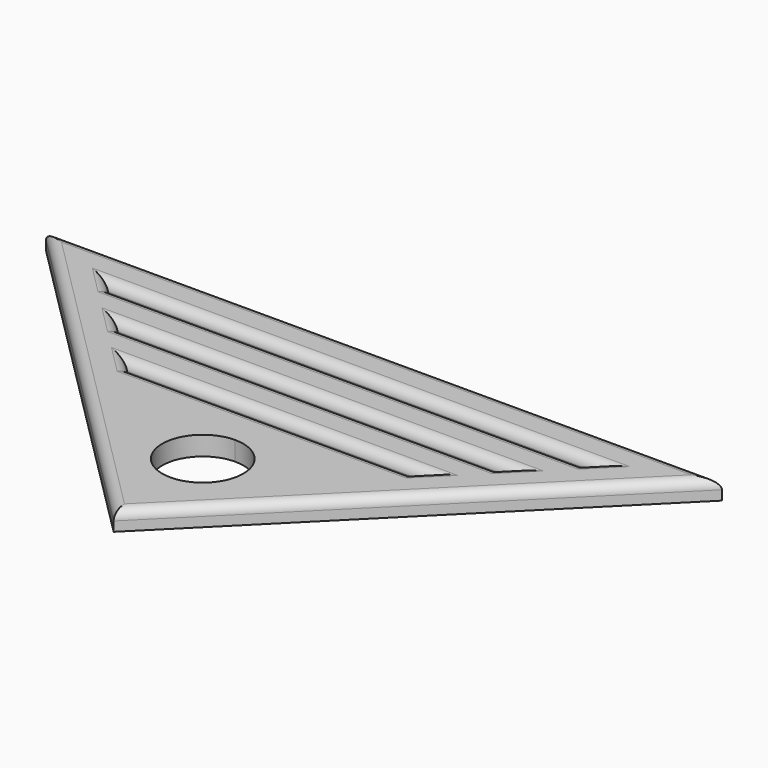
from build123d import *

# Parameters (mm, degrees)
F1_DEPTH = 4
F2_R     = 2
F3_R     = 1.99999


# Not quite as in the source:
# - a fillet or chamfer is up to 0.001 mm smaller than in the source, because OpenCascade refuses the exact size


with BuildPart() as f1:
    # F0 (on Top) → F1 (new body)
    with BuildSketch(Plane.XY):
        Polygon((-82.9944183651, 27.933470586), (-90.9944183651, 35.933470586), (-102.3081268641, 35.933470586), (-31.5974487455, -34.7772075326), (-31.5974487455, -23.4634990336), (-37.5931606391, -17.46778714), (-60.9944183651, 5.933470586), (-62.9944183651, 7.933470586), (-70.9944183651, 15.933470586), (-72.9944183651, 17.933470586), (-80.9944183651, 25.933470586), align=None)
        with BuildLine():
            Line((-60.9944183651, 5.933470586), (-37.5931606391, -17.46778714))
            ThreePointArc((-37.5931606391, -17.46778714), (-39.4312238538, -8.2272193518), (-31.5974487455, -2.9928581702))
            Line((-31.5974487455, -2.9928581702), (-31.5974487455, 5.933470586))
            Line((-31.5974487455, 5.933470586), (-60.9944183651, 5.933470586))
        make_face()
        with BuildLine():
            Line((-31.5974487455, -19.9512923224), (-31.5974487455, -23.4634990336))
            Line((-31.5974487455, -23.4634990336), (-25.6017368518, -17.46778714))
            ThreePointArc((-25.6017368518, -17.46778714), (-28.352592851, -19.3058503546), (-31.5974487455, -19.9512923224))
        make_face()
        Polygon((39.1132293732, 35.933470586), (27.7995208742, 35.933470586), (19.7995208742, 27.933470586), (17.7995208742, 25.933470586), (9.7995208742, 17.933470586), (7.7995208742, 15.933470586), (-0.2004791258, 7.933470586), (-2.2004791258, 5.933470586), (-25.6017368518, -17.46778714), (-31.5974487455, -23.4634990336), (-31.5974487455, -34.7772075326), align=None)
        with BuildLine():
            Line((-37.5931606391, -17.46778714), (-31.5974487455, -23.4634990336))
            Line((-31.5974487455, -23.4634990336), (-31.5974487455, -19.9512923224))
            ThreePointArc((-31.5974487455, -19.9512923224), (-34.8423046399, -19.3058503546), (-37.5931606391, -17.46778714))
        make_face()
        with BuildLine():
            ThreePointArc((-23.1182316693, -11.4720752463), (-23.7636736371, -14.7169311407), (-25.6017368518, -17.46778714))
            Line((-25.6017368518, -17.46778714), (-2.2004791258, 5.933470586))
            Line((-2.2004791258, 5.933470586), (-31.5974487455, 5.933470586))
            Line((-31.5974487455, 5.933470586), (-31.5974487455, -2.9928581702))
            ThreePointArc((-31.5974487455, -2.9928581702), (-25.6017368518, -5.4763633526), (-23.1182316693, -11.4720752463))
        make_face()
        Polygon((7.7995208742, 15.933470586), (-31.5974487455, 15.933470586), (-31.5974487455, 7.933470586), (-0.2004791258, 7.933470586), align=None)
        Polygon((-31.5974487455, 7.933470586), (-31.5974487455, 15.933470586), (-70.9944183651, 15.933470586), (-62.9944183651, 7.933470586), align=None)
        Polygon((17.7995208742, 25.933470586), (-31.5974487455, 25.933470586), (-31.5974487455, 17.933470586), (9.7995208742, 17.933470586), align=None)
        Polygon((-31.5974487455, 17.933470586), (-31.5974487455, 25.933470586), (-80.9944183651, 25.933470586), (-72.9944183651, 17.933470586), align=None)
        Polygon((27.7995208742, 35.933470586), (-31.5974487455, 35.933470586), (-31.5974487455, 27.933470586), (19.7995208742, 27.933470586), align=None)
        Polygon((-31.5974487455, 27.933470586), (-31.5974487455, 35.933470586), (-90.9944183651, 35.933470586), (-82.9944183651, 27.933470586), align=None)
    extrude(amount=F1_DEPTH)

    # F2
    f2_edges = [f1.edges().sort_by_distance(p)[0] for p in [
        (-31.597449, 35.933471, 4),
        (-31.597449, 27.933471, 4),
        (-31.597449, 25.933471, 4),
        (-31.597449, 17.933471, 4),
        (-31.597449, 15.933471, 4),
        (-31.597449, 7.933471, 4),
        (-31.597449, 5.933471, 4),
        (-66.952788, 0.578132, 4),
        (3.75789, 0.578132, 4),
        (8.799521, 16.933471, 4),
        (18.799521, 26.933471, 4),
        (-1.200479, 6.933471, 4),
        (-61.994418, 6.933471, 4),
        (-71.994418, 16.933471, 4),
        (-81.994418, 26.933471, 4),
    ]]
    fillet(f2_edges, radius=F2_R)

    # F3 (radius 2 in the source; OpenCascade refuses exactly that, so slightly less here)
    f3_edges = [f1.edges().sort_by_distance(p)[0] for p in [
        (-31.597449, 27.933471, 0),
        (-31.597449, 25.933471, 0),
        (-31.597449, 7.933471, 0),
        (-31.597449, 5.933471, 0),
        (-31.597449, 17.933471, 0),
        (-31.597449, 15.933471, 0),
    ]]
    fillet(f3_edges, radius=F3_R)


solid = f1.part
